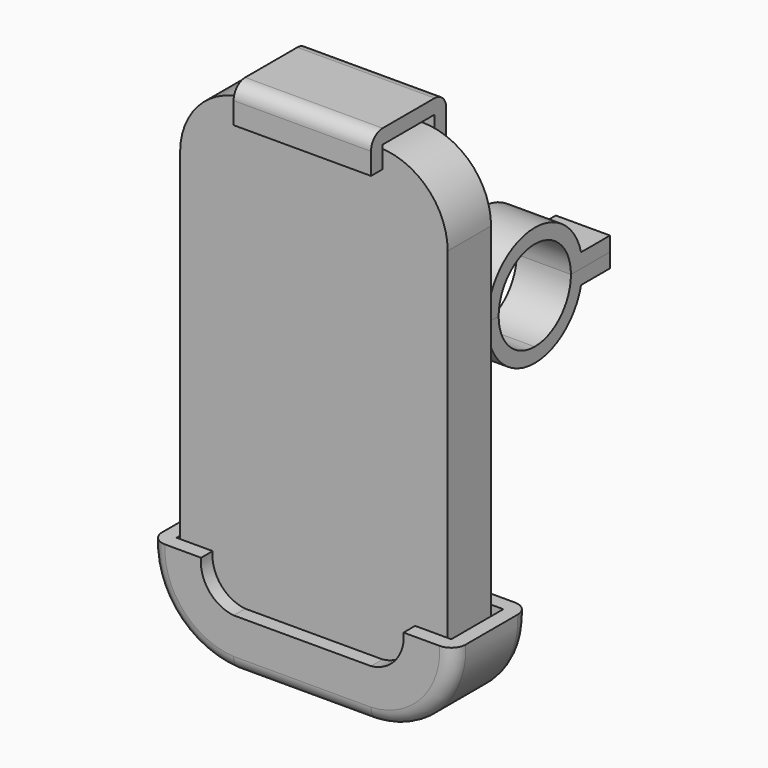
from build123d import *

# Parameters (mm, degrees)
F1_DEPTH     = 18
F2_T1_DEPTH  = 35.9
F2_T3_DEPTH  = 95.25
F2_T6_ANGLE  = 90
F2_T8_ANGLE  = 90
F2_T10_ANGLE = 90
F2_T12_ANGLE = 90
F4_DEPTH     = 19
F8_ANGLE     = 90
F12_DEPTH    = 4
F14_DEPTH    = 7.5
F15_DEPTH    = 7.5


# Not quite as in the source:
# - a fillet or chamfer that OpenCascade refuses, or shapes differently, is made with other operations: its cross-section is extruded or revolved along the edge and cut away or added


with BuildPart() as f1:
    # F0 (on Front) → F1 (new body)
    with BuildSketch(Plane.XZ):
        with BuildLine():
            Line((-17.95, -66.675), (17.95, -66.675))
            ThreePointArc((17.95, -66.675), (31.4203841816, -61.0953841816), (37, -47.625))
            Line((37, -47.625), (37, 47.625))
            ThreePointArc((37, 47.625), (31.4203841816, 61.0953841816), (17.95, 66.675))
            Line((17.95, 66.675), (-17.95, 66.675))
            ThreePointArc((-17.95, 66.675), (-31.4203841816, 61.0953841816), (-37, 47.625))
            Line((-37, 47.625), (-37, -47.625))
            ThreePointArc((-37, -47.625), (-31.4203841816, -61.0953841816), (-17.95, -66.675))
        make_face()
    extrude(amount=F1_DEPTH)

    # F2: chamfer of 15 x 3 on 8 edges, made by hand

    # F2_s2 → F2_t1 (cut)
    with BuildSketch(Plane.YZ.offset(-17.95)):
        Polygon((-3, -66.675), (0, -51.675), (0, -66.675), align=None)
        Polygon((-3, 66.675), (0, 51.675), (0, 66.675), align=None)
    extrude(amount=F2_T1_DEPTH, mode=Mode.SUBTRACT)

    # F2_s4 → F2_t3 (cut)
    with BuildSketch(Plane.XY.offset(-47.625)):
        Polygon((37, -3), (22, 0), (37, 0), align=None)
        Polygon((-37, -3), (-22, 0), (-37, 0), align=None)
    extrude(amount=F2_T3_DEPTH, mode=Mode.SUBTRACT)

    # F2_s5 → F2_t6 (revolve, cut)
    with BuildSketch(Plane.YZ.offset(17.95)):
        Polygon((-3, -66.675), (0, -51.675), (0, -66.675), align=None)
    revolve(axis=Axis((17.95, 0, -47.625), (0, -1, 0)), revolution_arc=F2_T6_ANGLE, mode=Mode.SUBTRACT)

    # F2_s7 → F2_t8 (revolve, cut)
    with BuildSketch(Plane.XY.offset(47.625)):
        Polygon((37, -3), (22, 0), (37, 0), align=None)
    revolve(axis=Axis((17.95, 0, 47.625), (0, -1, 0)), revolution_arc=F2_T8_ANGLE, mode=Mode.SUBTRACT)

    # F2_s9 → F2_t10 (revolve, cut)
    with BuildSketch(Plane.YZ.offset(-17.95)):
        Polygon((-3, 66.675), (0, 51.675), (0, 66.675), align=None)
    revolve(axis=Axis((-17.95, 0, 47.625), (0, -1, 0)), revolution_arc=F2_T10_ANGLE, mode=Mode.SUBTRACT)

    # F2_s11 → F2_t12 (revolve, cut)
    with BuildSketch(Plane.XY.offset(-47.625)):
        Polygon((-37, -3), (-22, 0), (-37, 0), align=None)
    revolve(axis=Axis((-17.95, 0, -47.625), (0, -1, 0)), revolution_arc=F2_T12_ANGLE, mode=Mode.SUBTRACT)


with BuildPart() as f4:
    # F3 (on Right) → F4 (new body, symmetric)
    with BuildSketch(Plane.YZ):
        with BuildLine():
            Line((-18, 66.675), (-18, 67.675))
            Line((-18, 67.675), (-1.4493813505, 67.675))
            Line((-1.4493813505, 67.675), (0, 67.675))
            Line((0, 67.675), (0, -67.675))
            Line((0, -67.675), (-18, -67.675))
            Line((-18, -67.675), (-18, -57.675))
            Line((-18, -57.675), (-22, -57.675))
            Line((-22, -57.675), (-22, -67.675))
            ThreePointArc((-22, -67.675), (-20.8284271247, -70.5034271247), (-18, -71.675))
            Line((-18, -71.675), (0, -71.675))
            ThreePointArc((0, -71.675), (2.8284271247, -70.5034271247), (4, -67.675))
            Line((4, -67.675), (4, 67.675))
            ThreePointArc((4, 67.675), (2.8284271247, 70.5034271247), (0, 71.675))
            Line((0, 71.675), (-18, 71.675))
            ThreePointArc((-18, 71.675), (-20.8284271247, 70.5034271247), (-22, 67.675))
            Line((-22, 67.675), (-22, 61.675))
            Line((-22, 61.675), (-18, 61.675))
            Line((-18, 61.675), (-18, 66.675))
        make_face()
    extrude(amount=F4_DEPTH, both=True)

    # F5 (on face) → F8 (revolve)
    with BuildSketch(Plane.YZ.offset(19)):
        with BuildLine():
            Line((0, -67.675), (-18, -67.675))
            Line((-18, -67.675), (-18, -57.675))
            Line((-18, -57.675), (-22, -57.675))
            Line((-22, -57.675), (-22, -67.675))
            ThreePointArc((-22, -67.675), (-20.8284271247, -70.5034271247), (-18, -71.675))
            Line((-18, -71.675), (0, -71.675))
            ThreePointArc((0, -71.675), (2.8284271247, -70.5034271247), (4, -67.675))
            Line((4, -67.675), (4, -57.675))
            Line((4, -57.675), (0, -57.675))
            Line((0, -57.675), (0, -67.675))
        make_face()
    revolve(axis=Axis((17.95, -13.3947152644, -47.625), (0, -1, 0)), revolution_arc=F8_ANGLE)


with BuildPart() as f9_1:
    # F9: instance of F4
    add(f4.part.mirror(Plane.YZ))

    # F10: union F4
    add(f4.part)

    # F11 (on face) → F12 (join)
    with BuildSketch(Plane(origin=(0, 4, 0), x_dir=(-1, 0, 0), z_dir=(0, 1, 0))):
        with BuildLine():
            Line((-19, -46.575), (-28, -46.575))
            ThreePointArc((-28, -46.575), (-25.7988852712, -53.9889610307), (-19, -57.675))
            Line((-19, -57.675), (-19, -46.575))
        make_face()
        with BuildLine():
            Line((28, -46.575), (19, -46.575))
            Line((19, -46.575), (19, -57.675))
            ThreePointArc((19, -57.675), (25.7988852712, -53.9889610307), (28, -46.575))
        make_face()
    extrude(amount=-F12_DEPTH)

    # F13 (on Right) → F14 (join, symmetric)
    with BuildSketch(Plane.YZ):
        with BuildLine():
            Line((0, 4), (0, 0))
            Line((0, 0), (22.9843788128, 0))
            Line((22.9843788128, 0), (36.4921894064, 0))
            ThreePointArc((36.4921894064, 0), (48.9921894064, 12.5), (61.4921894064, 0))
            Line((61.4921894064, 0), (75, 0))
            Line((75, 0), (75, 4))
            Line((75, 4), (65, 4))
            ThreePointArc((65, 4), (48.9921894064, 16.5), (32.9843788128, 4))
            Line((32.9843788128, 4), (0, 4))
        make_face()
    extrude(amount=F14_DEPTH, both=True)


with BuildPart() as f15:
    # F13 (on Right) → F15 (new body, symmetric)
    with BuildSketch(Plane.YZ):
        with BuildLine():
            Line((36.4921894064, 0), (22.9843788128, 0))
            Line((22.9843788128, 0), (22.9843788128, -4))
            Line((22.9843788128, -4), (32.9843788128, -4))
            ThreePointArc((32.9843788128, -4), (38.8371414006, -13.0048068036), (48.9921894064, -16.5))
            Line((48.9921894064, -16.5), (48.9921894064, -12.5))
            ThreePointArc((48.9921894064, -12.5), (40.1533546416, -8.8388347648), (36.4921894064, 0))
        make_face()
        with BuildLine():
            Line((75, 0), (61.4921894064, 0))
            ThreePointArc((61.4921894064, 0), (57.8310241712, -8.8388347648), (48.9921894064, -12.5))
            Line((48.9921894064, -12.5), (48.9921894064, -16.5))
            ThreePointArc((48.9921894064, -16.5), (59.1472374122, -13.0048068036), (65, -4))
            Line((65, -4), (75, -4))
            Line((75, -4), (75, 0))
        make_face()
    extrude(amount=F15_DEPTH, both=True)


solid = Compound([f1.part, f9_1.part, f15.part])
